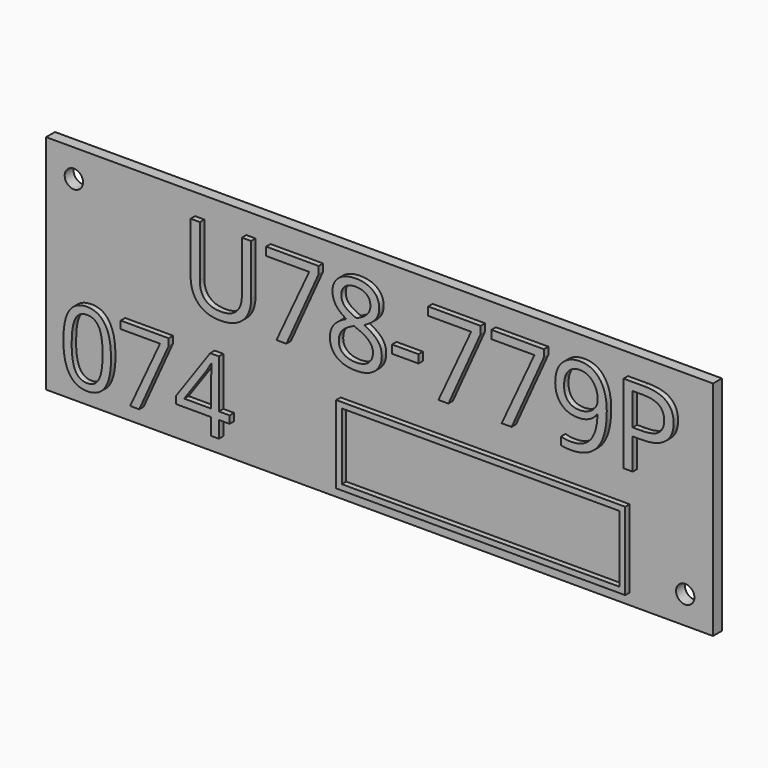
from build123d import *

# Parameters (mm, degrees)
F0_W         = 120
F0_H         = 40
F1_DEPTH     = 2
F3_D         = 3.3
F4_TEXT_SIZE = 19.8943114703
F5_DEPTH     = 1
F6_TEXT_SIZE = 18.1818181818
F7_DEPTH     = 1
F8_W         = 52
F8_H         = 14
F8_W_2       = 49.99999962
F8_H_2       = 11.99999962
F9_DEPTH     = 1


# Not quite as in the source:
# - Text() gives the source's letters only with a copy of the font that has no kerning and outlines rounded to 1/6400 em; it was checked with that copy


with BuildPart() as f1:
    # F0 (on Front) → F1 (new body)
    with BuildSketch(Plane.XZ):
        Rectangle(F0_W, F0_H)
    extrude(amount=F1_DEPTH)

    # F3 (through all)
    with Locations(Plane.XZ.offset(2)):
        with Locations((-55, 15), (55, -15)):
            Hole(F3_D / 2)

    # F4 (on face) → F5 (join)
    with BuildSketch(Plane.XZ.offset(2)):
        with Locations((-35, 2)):
            Text('U78-779P', F4_TEXT_SIZE, font='Open Sans', text_align=(TextAlign.LEFT, TextAlign.BOTTOM))
    extrude(amount=F5_DEPTH)

    # F6 (on face) → F7 (join)
    with BuildSketch(Plane.XZ.offset(2)):
        with Locations((-57, -17)):
            Text('074', F6_TEXT_SIZE, font='Open Sans', text_align=(TextAlign.LEFT, TextAlign.BOTTOM))
    extrude(amount=F7_DEPTH)

    # F8 (on face) → F9 (join)
    with BuildSketch(Plane.XZ.offset(2)):
        with Locations((19, -11)):
            Rectangle(F8_W, F8_H)
        with Locations((19, -11)):
            Rectangle(F8_W_2, F8_H_2, mode=Mode.SUBTRACT)
    extrude(amount=F9_DEPTH)


solid = f1.part
